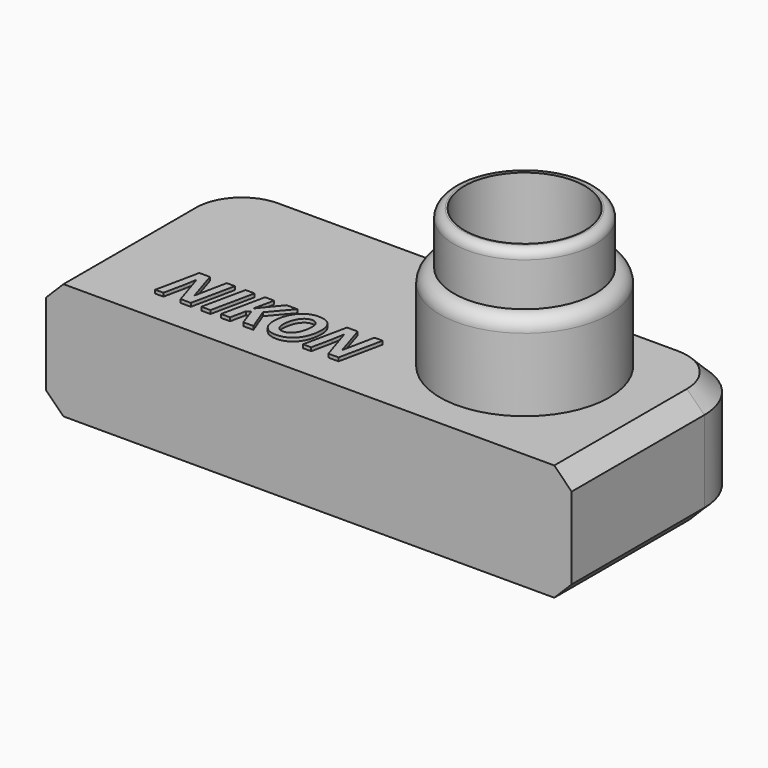
from build123d import *

# Parameters (mm, degrees)
F0_W          = 151.1903554201
F0_H          = 65.8338814974
F1_DEPTH      = 33.5
F2_R          = 24.3707690354
F3_DEPTH      = 25
F4_R          = 18.1066017178
F5_R          = 18.107
F6_SIZE       = 5
F8_W          = 66.4495043457
F8_H          = 34.2659512535
F9_DEPTH      = 1
F10_R         = 4
F11_R         = 20.3500467872
F12_DEPTH     = 15
F13_R         = 2.5
F14_R         = 17.3291986396
F15_DEPTH     = 41.1
F17_R         = 7.3430812258
F18_DEPTH     = 1.5
F19_W         = 10.7617210597
F19_H         = 25.7662367076
F20_DEPTH     = 1.1
F21_W         = 25.9385565296
F21_H         = 8.9194718748
F22_DEPTH     = 1
F23_R         = 6.1040685909
F24_DEPTH     = 2.2
F25_TEXT_SIZE = 17.5666749581
F26_DEPTH     = 1


# Not quite as in the source:
# - Text() gives the source's letters only with a copy of the font that has no kerning and outlines rounded to 1/6400 em; it was checked with that copy


with BuildPart() as f1:
    # F0 (on Top) → F1 (new body)
    with BuildSketch(Plane.XY):
        with Locations((75.5951777101, 32.9169407487)):
            Rectangle(F0_W, F0_H)
    extrude(amount=F1_DEPTH)

    # F2 (on face) → F3 (join)
    with BuildSketch(Plane.XY.offset(33.5)):
        with Locations((110.8216866851, 33.5641242564)):
            Circle(F2_R)
    extrude(amount=F3_DEPTH)

    # F4
    f4_edges = [f1.edges().sort_by_distance(p)[0] for p in [
        (151.190355, 65.833881, 16.75),
    ]]
    fillet(f4_edges, radius=F4_R)

    # F5
    f5_edges = [f1.edges().sort_by_distance(p)[0] for p in [
        (0, 65.833881, 16.75),
    ]]
    fillet(f5_edges, radius=F5_R)

    # F6
    f6_edges = [f1.edges().sort_by_distance(p)[0] for p in [
        (151.190355, 23.86364, 33.5),
        (145.887055, 60.530581, 33.5),
        (75.595377, 65.833881, 33.5),
        (5.303418, 60.530464, 33.5),
        (0, 23.863441, 33.5),
        (151.190355, 23.86364, 0),
        (145.887055, 60.530581, 0),
        (75.595377, 65.833881, 0),
        (0, 23.863441, 0),
        (5.303418, 60.530464, 0),
    ]]
    chamfer(f6_edges, length=F6_SIZE)

    # F8 (on face) → F9 (cut)
    with BuildSketch(Plane(origin=(0, 0, 0), x_dir=(1, 0, 0), z_dir=(0, 0, -1))):
        with Locations((73.4730381519, -28.1266192906)):
            Rectangle(F8_W, F8_H)
    extrude(amount=-F9_DEPTH, mode=Mode.SUBTRACT)

    # F10
    f10_edges = [f1.edges().sort_by_distance(p)[0] for p in [
        (86.450918, 33.564124, 58.5),
    ]]
    fillet(f10_edges, radius=F10_R)

    # F11 (on face) → F12 (join)
    with BuildSketch(Plane.XY.offset(58.5)):
        with Locations((110.8216866851, 33.5641242564)):
            Circle(F11_R)
    extrude(amount=F12_DEPTH)

    # F13
    f13_edges = [f1.edges().sort_by_distance(p)[0] for p in [
        (90.47164, 33.564124, 73.5),
    ]]
    fillet(f13_edges, radius=F13_R)

    # F14 (on face) → F15 (cut)
    with BuildSketch(Plane.XY.offset(73.5)):
        with Locations((110.8216866851, 33.5641242564)):
            Circle(F14_R)
    extrude(amount=-F15_DEPTH, mode=Mode.SUBTRACT)

    # F17 (on face) → F18 (join)
    with BuildSketch(Plane(origin=(0, 0, 0), x_dir=(1, 0, 0), z_dir=(0, 0, -1))):
        with Locations((127.0308345556, -44.2757979035)):
            Circle(F17_R)
    extrude(amount=F18_DEPTH)

    # F19 (on face) → F20 (join)
    with BuildSketch(Plane(origin=(0, 0, 0), x_dir=(1, 0, 0), z_dir=(0, 0, -1))):
        with Locations((19.2668521777, -33.302613534)):
            Rectangle(F19_W, F19_H)
    extrude(amount=F20_DEPTH)

    # F21 (on face) → F22 (join)
    with BuildSketch(Plane(origin=(0, 0, 0), x_dir=(1, 0, 0), z_dir=(0, 0, -1))):
        with Locations((19.5716838352, -31.7770196125)):
            Rectangle(F21_W, F21_H)
    extrude(amount=F22_DEPTH)

    # F23 (on face) → F24 (join)
    with BuildSketch(Plane(origin=(0, 65.8338814974, 0), x_dir=(-1, 0, 0), z_dir=(0, 1, 0))):
        with Locations((-35.5104021728, 16.6898779571)):
            Circle(F23_R)
    extrude(amount=F24_DEPTH)

    # F25 (on face) → F26 (join)
    with BuildSketch(Plane.XY.offset(33.5)):
        with Locations((23.5296506435, 9.2715034261)):
            Text('NIKON', F25_TEXT_SIZE, font='Open Sans', font_style=FontStyle.BOLDITALIC, text_align=(TextAlign.LEFT, TextAlign.BOTTOM))
    extrude(amount=F26_DEPTH)


solid = f1.part
